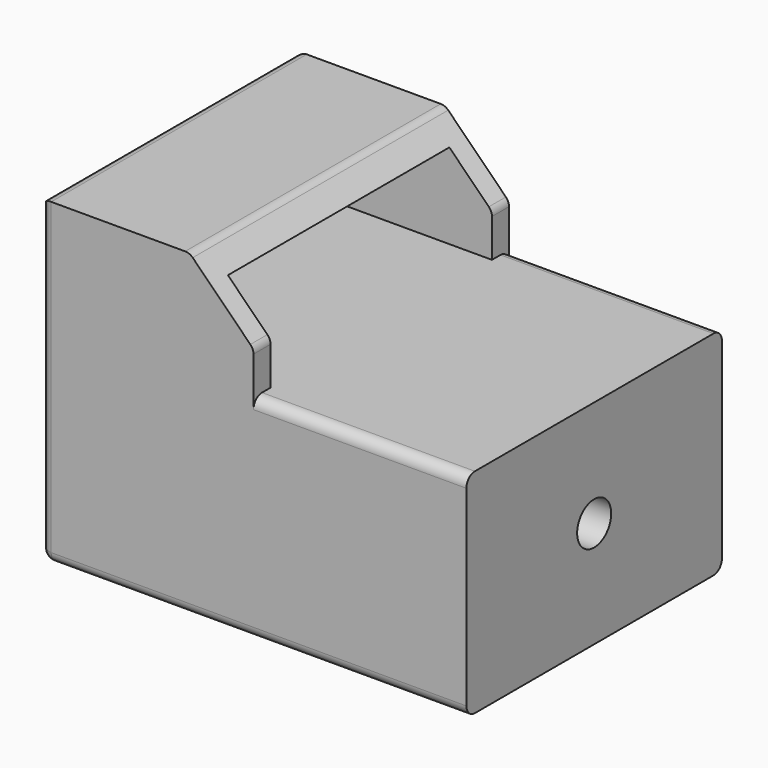
from build123d import *

# Parameters (mm, degrees)
F0_W      = 200
F0_H      = 150
F0_R      = 10
F1_DEPTH  = 100
F2_DEPTH  = 20
F3_W      = 100
F3_H      = 10
F4_DEPTH  = 50
F5_SIZE   = 30
F6_W      = 70
F6_H      = 10
F7_DEPTH  = 130
F8_R      = 4.99999
F9_R      = 10
F10_DEPTH = 20


# Not quite as in the source:
# - a fillet or chamfer is up to 0.001 mm smaller than in the source, because OpenCascade refuses the exact size


with BuildPart() as f1:
    # F0 (on Top) → F1 (new body)
    with BuildSketch(Plane.XY):
        with Locations((-14.7118499619, 7.1657538414)):
            Rectangle(F0_W, F0_H)
        with Locations((-14.7118499619, 7.1657538414)):
            Circle(F0_R, mode=Mode.SUBTRACT)
        with Locations((-14.7118499619, 7.1657538414)):
            Circle(F0_R)
    extrude(amount=F1_DEPTH)

    # F0 (on Top) → F2 (join)
    with BuildSketch(Plane.XY):
        with Locations((-14.7118499619, 7.1657538414)):
            Circle(F0_R)
    extrude(amount=-F2_DEPTH)

    # F3 (on face) → F4 (join)
    with BuildSketch(Plane.XY.offset(100)):
        with Locations((-64.7118499619, 77.1657538414)):
            Rectangle(F3_W, F3_H)
        with Locations((-64.7118499619, -62.8342461586)):
            Rectangle(F3_W, F3_H)
    extrude(amount=F4_DEPTH)

    # F5
    f5_edges = [f1.edges().sort_by_distance(p)[0] for p in [
        (-14.71185, -62.834246, 150),
        (-14.71185, 77.165754, 150),
    ]]
    chamfer(f5_edges, length=F5_SIZE)

    # F6 (on face) → F7 (join)
    with BuildSketch(Plane.XZ.offset(-72.1657538414)):
        with Locations((-79.7118499619, 145)):
            Rectangle(F6_W, F6_H)
        Polygon((-34.7118499619, 140), (-44.7118499619, 150), (-44.7118499619, 140), align=None)
    extrude(amount=F7_DEPTH)

    # F8 (radius 5 in the source; OpenCascade refuses exactly that, so slightly less here)
    f8_edges = [f1.edges().sort_by_distance(p)[0] for p in [
        (35.28815, 82.165754, 100),
        (35.28815, -67.834246, 100),
        (-14.71185, 82.165754, 0),
        (-14.71185, -67.834246, 0),
        (-114.71185, 82.165754, 75),
        (-114.71185, 7.165754, 150),
        (-114.71185, -67.834246, 75),
        (-114.71185, 7.165754, 0),
        (-114.71185, 72.165754, 120),
        (-114.71185, 7.165754, 100),
        (-114.71185, -57.834246, 120),
        (-114.71185, 7.165754, 140),
        (-14.71185, -62.834246, 120),
        (-44.71185, 7.165754, 150),
        (-14.71185, 77.165754, 120),
    ]]
    fillet(f8_edges, radius=F8_R)

    # F9 (on face) → F10 (cut)
    with BuildSketch(Plane.YZ.offset(85.2881500381)):
        with Locations((7.1657538414, 50)):
            Circle(F9_R)
    extrude(amount=-F10_DEPTH, mode=Mode.SUBTRACT)


solid = f1.part
